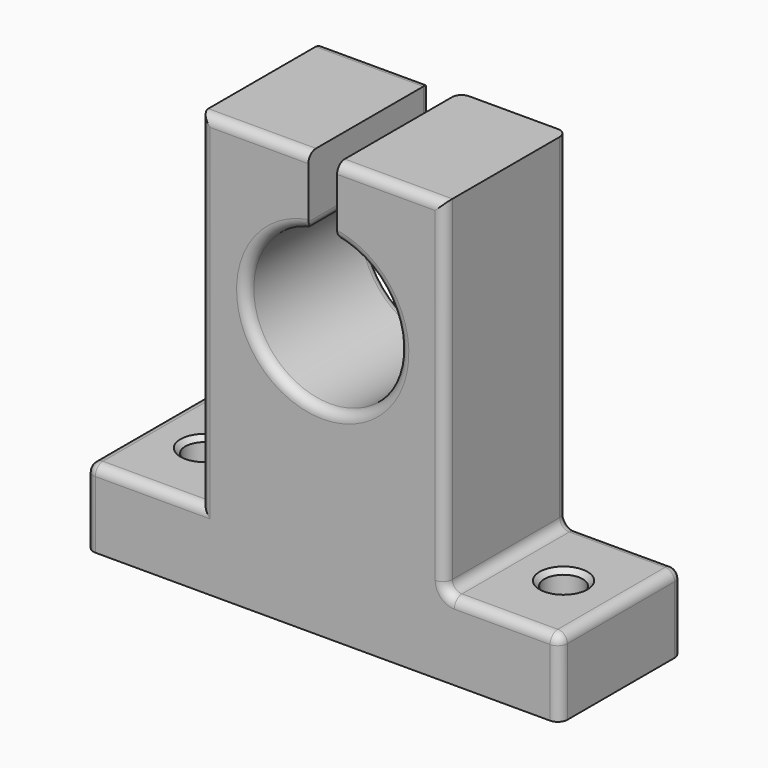
from build123d import *

# Parameters (mm, degrees)
F1_DEPTH       = 8
F3_D           = 4
F3_CSINK_D     = 5
F3_CSINK_ANGLE = 90
F4_R           = 1


with BuildPart() as f1:
    # F0 (on Front) → F1 (new body, symmetric)
    with BuildSketch(Plane.XZ):
        with BuildLine():
            Line((0, -5.3220339234), (24.75, -5.3220339234))
            Line((24.75, -5.3220339234), (24.75, 2.6779660766))
            Line((24.75, 2.6779660766), (12.75, 2.6779660766))
            Line((12.75, 2.6779660766), (12.75, 38.6779660766))
            Line((12.75, 38.6779660766), (1.5, 38.6779660766))
            Line((1.5, 38.6779660766), (1.5, 31.5360828994))
            ThreePointArc((1.5, 31.5360828994), (7.964450219, 22.9246184085), (0, 15.6779660766))
            Line((0, 15.6779660766), (0, -5.3220339234))
        make_face()
        with BuildLine():
            Line((-24.75, -5.3220339234), (0, -5.3220339234))
            Line((0, -5.3220339234), (0, 15.6779660766))
            ThreePointArc((0, 15.6779660766), (-7.964450219, 22.9246184085), (-1.5, 31.5360828994))
            Line((-1.5, 31.5360828994), (-1.5, 38.6779660766))
            Line((-1.5, 38.6779660766), (-12.75, 38.6779660766))
            Line((-12.75, 38.6779660766), (-12.75, 2.6779660766))
            Line((-12.75, 2.6779660766), (-24.75, 2.6779660766))
            Line((-24.75, 2.6779660766), (-24.75, -5.3220339234))
        make_face()
    extrude(amount=F1_DEPTH, both=True)

    # F3 (through all)
    with Locations(Plane.XY.offset(2.6779660766)):
        with Locations((18.75, 0), (-18.75, 0)):
            CounterSinkHole(F3_D / 2, F3_CSINK_D / 2, counter_sink_angle=F3_CSINK_ANGLE)

    # F4
    f4_edges = [f1.edges().sort_by_distance(p)[0] for p in [
        (-12.75, -8, 20.677966),
        (-7.125, -8, 38.677966),
        (7.125, -8, 38.677966),
        (12.75, -8, 20.677966),
        (18.75, -8, 2.677966),
        (-18.75, -8, 2.677966),
        (24.75, -8, -1.322034),
        (-24.75, -8, -1.322034),
        (12.75, 0, 2.677966),
        (24.75, 0, 2.677966),
        (24.75, 8, -1.322034),
        (12.75, 8, 20.677966),
        (1.5, 8, 35.107024),
        (-1.5, 8, 35.107024),
        (1.5, 0, 31.536083),
        (0, 8, 15.677966),
        (-1.5, 0, 31.536083),
        (0, -8, 15.677966),
        (-7.125, 8, 38.677966),
        (-12.75, 8, 20.677966),
        (-18.75, 8, 2.677966),
        (-24.75, 8, -1.322034),
        (-24.75, 0, 2.677966),
        (18.75, 8, 2.677966),
    ]]
    fillet(f4_edges, radius=F4_R)


solid = f1.part
